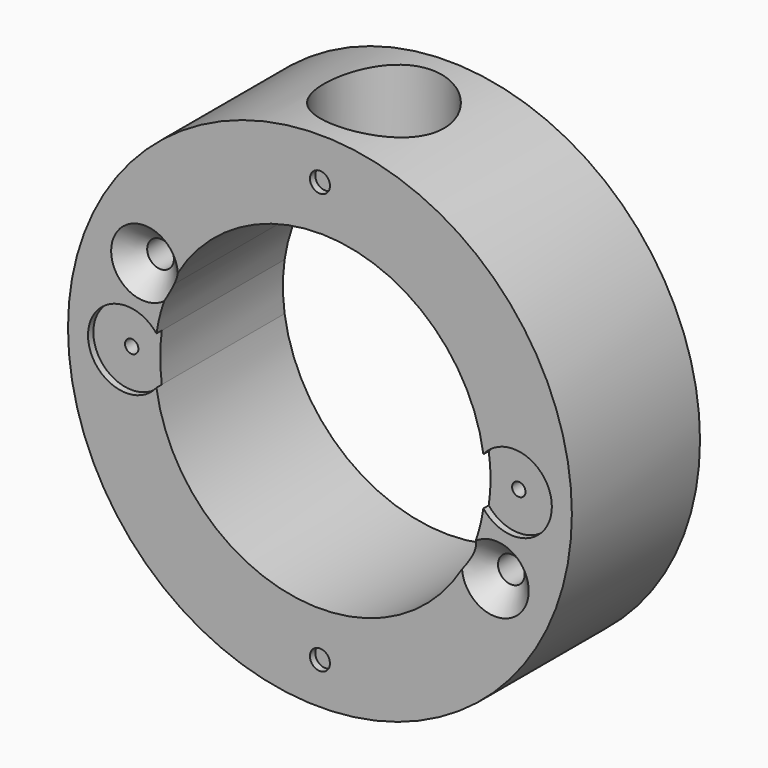
from build123d import *

# Parameters (mm, degrees)
F0_R     = 37.75
F0_R_2   = 1.5
F0_R_3   = 2
F1_DEPTH = 24
F0_R_4   = 1
F2_DEPTH = 23
F5_R     = 9
F5_R_2   = 8
F6_DEPTH = 25
F7_DEPTH = 15


# Not quite as in the source:
# - a fillet or chamfer that OpenCascade refuses, or shapes differently, is made with other operations: its cross-section is extruded or revolved along the edge and cut away or added


with BuildPart() as f1:
    # F0 (on Front) → F1 (new body)
    with BuildSketch(Plane.XZ):
        Circle(F0_R)
        with Locations((0, -31.5)):
            Circle(F0_R_2, mode=Mode.SUBTRACT)
        with Locations((26.2829258241, -12.2559295905)):
            Circle(F0_R_3, mode=Mode.SUBTRACT)
        with BuildLine():
            ThreePointArc((-24.2829258241, 12.2559295905), (-24.3303338098, 11.8230503626), (-24.47031025, 11.410693067))
            ThreePointArc((-24.47031025, 11.410693067), (-28.2355178383, 12.6888088184), (-24.2829258241, 12.2559295905))
        make_face(mode=Mode.SUBTRACT)
        with BuildLine():
            ThreePointArc((10.4598019781, 22.4311177292), (19.8581217638, 14.7721867038), (24.4913793103, 3.568590685))
            ThreePointArc((24.4913793103, 3.568590685), (30.8891705898, 5.4307950139), (34.75, 0))
            ThreePointArc((34.75, 0), (30.8891705898, -5.4307950139), (24.4913793103, -3.568590685))
            ThreePointArc((24.4913793103, -3.568590685), (0, -24.75), (-24.4913793103, -3.568590685))
            ThreePointArc((-24.4913793103, -3.568590685), (-34.75, 0), (-24.4913793103, 3.568590685))
            ThreePointArc((-24.4913793103, 3.568590685), (-23.7129158978, 7.0894371866), (-22.4311177292, 10.4598019781))
            ThreePointArc((-22.4311177292, 10.4598019781), (-8.4649985473, 23.2573923645), (10.4598019781, 22.4311177292))
        make_face(mode=Mode.SUBTRACT)
        with Locations((0, 31.5)):
            Circle(F0_R_2, mode=Mode.SUBTRACT)
    extrude(amount=F1_DEPTH)

    # F0 (on Front) → F2 (join)
    with BuildSketch(Plane.XZ):
        with BuildLine():
            ThreePointArc((-24.4913793103, 3.568590685), (-34.75, 0), (-24.4913793103, -3.568590685))
            ThreePointArc((-24.4913793103, -3.568590685), (-24.75, 0), (-24.4913793103, 3.568590685))
        make_face()
        with Locations((-29, 0)):
            Circle(F0_R_4, mode=Mode.SUBTRACT)
        with Locations((0, 31.5)):
            Circle(F0_R_2)
        with BuildLine():
            ThreePointArc((24.4913793103, 3.568590685), (24.6852601559, 1.7889748557), (24.75, 0))
            ThreePointArc((24.75, 0), (24.6852601559, -1.7889748557), (24.4913793103, -3.568590685))
            ThreePointArc((24.4913793103, -3.568590685), (30.8891705898, -5.4307950139), (34.75, 0))
            ThreePointArc((34.75, 0), (30.8891705898, 5.4307950139), (24.4913793103, 3.568590685))
        make_face()
        with Locations((29, 0)):
            Circle(F0_R_4, mode=Mode.SUBTRACT)
        with Locations((0, -31.5)):
            Circle(F0_R_2)
    extrude(amount=F2_DEPTH)

    # F3: chamfer of 3 on 2 edges, made by hand

    # F3_s1 → F3_t2 (revolve, cut)
    with BuildSketch(Plane.XY.offset(12.2559295905)):
        Polygon((-21.2829258241, -24), (-24.2829258241, -21), (-24.2829258241, -24), align=None)
    revolve(axis=Axis((-26.2829258241, -24, 12.2559295905), (0, -1, 0)), mode=Mode.SUBTRACT)

    # F3_s3 → F3_t4 (revolve, cut)
    with BuildSketch(Plane.XY.offset(-12.2559295905)):
        Polygon((31.2829258241, -24), (28.2829258241, -21), (28.2829258241, -24), align=None)
    revolve(axis=Axis((26.2829258241, -24, -12.2559295905), (0, -1, 0)), mode=Mode.SUBTRACT)

    # F5 (on offset) → F6 (cut)
    with BuildSketch(Plane.XY.offset(26.25)):
        with Locations((0, -12)):
            Circle(F5_R)
        with Locations((0, -12)):
            Circle(F5_R_2, mode=Mode.SUBTRACT)
    extrude(amount=F6_DEPTH, mode=Mode.SUBTRACT)

    # F5 (on offset) → F7 (cut, symmetric)
    with BuildSketch(Plane.XY.offset(26.25)):
        with Locations((0, -12)):
            Circle(F5_R_2)
    extrude(amount=F7_DEPTH, both=True, mode=Mode.SUBTRACT)


solid = f1.part
